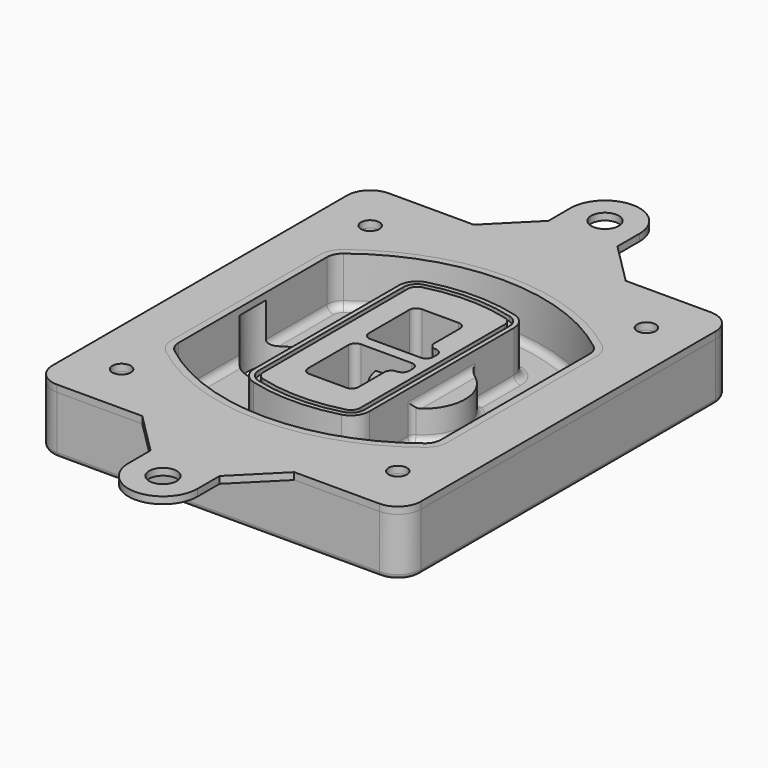
from build123d import *

# Parameters (mm, degrees)
F0_R      = 4
F1_DEPTH  = 25
F2_DEPTH  = 3
F3_DEPTH  = 18
F5_DEPTH  = 21
F6_DEPTH  = 2
F8_DEPTH  = 20
F9_DEPTH  = 16
F10_DEPTH = 25
F7_R      = 6
F7_R_2    = 4
F11_DEPTH = 6
F13_DEPTH = 9
F14_R     = 3
F15_R     = 2
F16_R     = 6
F16_R_2   = 4
F17_DEPTH = 3


# Not quite as in the source:
# - a feature names something its author has since deleted; it is built from what else it names


with BuildPart() as f1:
    # F0 (on Top) → F1 (new body)
    with BuildSketch(Plane.XY):
        with BuildLine():
            ThreePointArc((-80, -80), (-77.0710678119, -87.0710678119), (-70, -90))
            Line((-70, -90), (70, -90))
            ThreePointArc((70, -90), (77.0710678119, -87.0710678119), (80, -80))
            Line((80, -80), (80, 80))
            ThreePointArc((80, 80), (77.0710678119, 87.0710678119), (70, 90))
            Line((70, 90), (-70, 90))
            ThreePointArc((-70, 90), (-77.0710678119, 87.0710678119), (-80, 80))
            Line((-80, 80), (-80, -80))
        make_face()
        with Locations((-60, -67.5)):
            Circle(F0_R, mode=Mode.SUBTRACT)
        with Locations((60, -67.5)):
            Circle(F0_R, mode=Mode.SUBTRACT)
        with Locations((-60, 67.5)):
            Circle(F0_R, mode=Mode.SUBTRACT)
        with BuildLine():
            ThreePointArc((-64, 40.2934422872), (-62.5820384798, 46.4328484224), (-58.6153846154, 51.3286200352))
            ThreePointArc((-58.6153846154, 51.3286200352), (0, 71.5), (58.6153846154, 51.3286200352))
            ThreePointArc((58.6153846154, 51.3286200352), (62.5820384798, 46.4328484224), (64, 40.2934422872))
            Line((64, 40.2934422872), (64, -40.2934422872))
            ThreePointArc((64, -40.2934422872), (62.5820384798, -46.4328484224), (58.6153846154, -51.3286200352))
            ThreePointArc((58.6153846154, -51.3286200352), (0, -71.5), (-58.6153846154, -51.3286200352))
            ThreePointArc((-58.6153846154, -51.3286200352), (-62.5820384798, -46.4328484224), (-64, -40.2934422872))
            Line((-64, -40.2934422872), (-64, 40.2934422872))
        make_face(mode=Mode.SUBTRACT)
        with Locations((60, 67.5)):
            Circle(F0_R, mode=Mode.SUBTRACT)
        with BuildLine():
            ThreePointArc((58.6153846154, 51.3286200352), (0, 71.5), (-58.6153846154, 51.3286200352))
            ThreePointArc((-58.6153846154, 51.3286200352), (-62.5820384798, 46.4328484224), (-64, 40.2934422872))
            Line((-64, 40.2934422872), (-64, -40.2934422872))
            ThreePointArc((-64, -40.2934422872), (-62.5820384798, -46.4328484224), (-58.6153846154, -51.3286200352))
            ThreePointArc((-58.6153846154, -51.3286200352), (0, -71.5), (58.6153846154, -51.3286200352))
            ThreePointArc((58.6153846154, -51.3286200352), (62.5820384798, -46.4328484224), (64, -40.2934422872))
            Line((64, -40.2934422872), (64, 40.2934422872))
            ThreePointArc((64, 40.2934422872), (62.5820384798, 46.4328484224), (58.6153846154, 51.3286200352))
        make_face()
        with BuildLine():
            Line((-60, -40.2934422872), (-60, 40.2934422872))
            ThreePointArc((-60, 40.2934422872), (-58.9871703427, 44.6787323838), (-56.1538461538, 48.1757121072))
            ThreePointArc((-56.1538461538, 48.1757121072), (0, 67.5), (56.1538461538, 48.1757121072))
            ThreePointArc((56.1538461538, 48.1757121072), (58.9871703427, 44.6787323838), (60, 40.2934422872))
            Line((60, 40.2934422872), (60, -40.2934422872))
            ThreePointArc((60, -40.2934422872), (58.9871703427, -44.6787323838), (56.1538461538, -48.1757121072))
            ThreePointArc((56.1538461538, -48.1757121072), (0, -67.5), (-56.1538461538, -48.1757121072))
            ThreePointArc((-56.1538461538, -48.1757121072), (-58.9871703427, -44.6787323838), (-60, -40.2934422872))
        make_face(mode=Mode.SUBTRACT)
        with BuildLine():
            ThreePointArc((-56.1538461538, 48.1757121072), (-58.9871703427, 44.6787323838), (-60, 40.2934422872))
            Line((-60, 40.2934422872), (-60, -40.2934422872))
            ThreePointArc((-60, -40.2934422872), (-58.9871703427, -44.6787323838), (-56.1538461538, -48.1757121072))
            ThreePointArc((-56.1538461538, -48.1757121072), (0, -67.5), (56.1538461538, -48.1757121072))
            ThreePointArc((56.1538461538, -48.1757121072), (58.9871703427, -44.6787323838), (60, -40.2934422872))
            Line((60, -40.2934422872), (60, 40.2934422872))
            ThreePointArc((60, 40.2934422872), (58.9871703427, 44.6787323838), (56.1538461538, 48.1757121072))
            ThreePointArc((56.1538461538, 48.1757121072), (0, 67.5), (-56.1538461538, 48.1757121072))
        make_face()
        with BuildLine():
            ThreePointArc((54.3076923077, 45.8110311612), (56.2910192399, 43.3631453548), (57, 40.2934422872))
            Line((57, 40.2934422872), (57, -40.2934422872))
            ThreePointArc((57, -40.2934422872), (56.2910192399, -43.3631453548), (54.3076923077, -45.8110311612))
            ThreePointArc((54.3076923077, -45.8110311612), (0, -64.5), (-54.3076923077, -45.8110311612))
            ThreePointArc((-54.3076923077, -45.8110311612), (-56.2910192399, -43.3631453548), (-57, -40.2934422872))
            Line((-57, -40.2934422872), (-57, 40.2934422872))
            ThreePointArc((-57, 40.2934422872), (-56.2910192399, 43.3631453548), (-54.3076923077, 45.8110311612))
            ThreePointArc((-54.3076923077, 45.8110311612), (0, 64.5), (54.3076923077, 45.8110311612))
        make_face(mode=Mode.SUBTRACT)
        with BuildLine():
            Line((57, -40.2934422872), (57, 40.2934422872))
            ThreePointArc((57, 40.2934422872), (56.2910192399, 43.3631453548), (54.3076923077, 45.8110311612))
            ThreePointArc((54.3076923077, 45.8110311612), (0, 64.5), (-54.3076923077, 45.8110311612))
            ThreePointArc((-54.3076923077, 45.8110311612), (-56.2910192399, 43.3631453548), (-57, 40.2934422872))
            Line((-57, 40.2934422872), (-57, -40.2934422872))
            ThreePointArc((-57, -40.2934422872), (-56.2910192399, -43.3631453548), (-54.3076923077, -45.8110311612))
            ThreePointArc((-54.3076923077, -45.8110311612), (0, -64.5), (54.3076923077, -45.8110311612))
            ThreePointArc((54.3076923077, -45.8110311612), (56.2910192399, -43.3631453548), (57, -40.2934422872))
        make_face()
    extrude(amount=-F1_DEPTH)

    # F0 (on Top) → F2 (join)
    with BuildSketch(Plane.XY):
        with BuildLine():
            ThreePointArc((-56.1538461538, 48.1757121072), (-58.9871703427, 44.6787323838), (-60, 40.2934422872))
            Line((-60, 40.2934422872), (-60, -40.2934422872))
            ThreePointArc((-60, -40.2934422872), (-58.9871703427, -44.6787323838), (-56.1538461538, -48.1757121072))
            ThreePointArc((-56.1538461538, -48.1757121072), (0, -67.5), (56.1538461538, -48.1757121072))
            ThreePointArc((56.1538461538, -48.1757121072), (58.9871703427, -44.6787323838), (60, -40.2934422872))
            Line((60, -40.2934422872), (60, 40.2934422872))
            ThreePointArc((60, 40.2934422872), (58.9871703427, 44.6787323838), (56.1538461538, 48.1757121072))
            ThreePointArc((56.1538461538, 48.1757121072), (0, 67.5), (-56.1538461538, 48.1757121072))
        make_face()
        with BuildLine():
            ThreePointArc((54.3076923077, 45.8110311612), (56.2910192399, 43.3631453548), (57, 40.2934422872))
            Line((57, 40.2934422872), (57, -40.2934422872))
            ThreePointArc((57, -40.2934422872), (56.2910192399, -43.3631453548), (54.3076923077, -45.8110311612))
            ThreePointArc((54.3076923077, -45.8110311612), (0, -64.5), (-54.3076923077, -45.8110311612))
            ThreePointArc((-54.3076923077, -45.8110311612), (-56.2910192399, -43.3631453548), (-57, -40.2934422872))
            Line((-57, -40.2934422872), (-57, 40.2934422872))
            ThreePointArc((-57, 40.2934422872), (-56.2910192399, 43.3631453548), (-54.3076923077, 45.8110311612))
            ThreePointArc((-54.3076923077, 45.8110311612), (0, 64.5), (54.3076923077, 45.8110311612))
        make_face(mode=Mode.SUBTRACT)
    extrude(amount=F2_DEPTH)

    # F0 (on Top) → F3 (cut)
    with BuildSketch(Plane.XY):
        with BuildLine():
            Line((57, -40.2934422872), (57, 40.2934422872))
            ThreePointArc((57, 40.2934422872), (56.2910192399, 43.3631453548), (54.3076923077, 45.8110311612))
            ThreePointArc((54.3076923077, 45.8110311612), (0, 64.5), (-54.3076923077, 45.8110311612))
            ThreePointArc((-54.3076923077, 45.8110311612), (-56.2910192399, 43.3631453548), (-57, 40.2934422872))
            Line((-57, 40.2934422872), (-57, -40.2934422872))
            ThreePointArc((-57, -40.2934422872), (-56.2910192399, -43.3631453548), (-54.3076923077, -45.8110311612))
            ThreePointArc((-54.3076923077, -45.8110311612), (0, -64.5), (54.3076923077, -45.8110311612))
            ThreePointArc((54.3076923077, -45.8110311612), (56.2910192399, -43.3631453548), (57, -40.2934422872))
        make_face()
    extrude(amount=-F3_DEPTH, mode=Mode.SUBTRACT)

    # F4 (on face) → F5 (join, through all)
    with BuildSketch(Plane.XY.offset(3)):
        with BuildLine():
            ThreePointArc((-25, -39.2465276821), (-23.3511545998, -44.1109737193), (-19.0842911877, -46.9702398883))
            ThreePointArc((-19.0842911877, -46.9702398883), (0, -49.5), (19.0842911877, -46.9702398883))
            ThreePointArc((19.0842911877, -46.9702398883), (23.3511545998, -44.1109737193), (25, -39.2465276821))
            Line((25, -39.2465276821), (25, 39.2465276821))
            ThreePointArc((25, 39.2465276821), (23.3511545998, 44.1109737193), (19.0842911877, 46.9702398883))
            ThreePointArc((19.0842911877, 46.9702398883), (0, 49.5), (-19.0842911877, 46.9702398883))
            ThreePointArc((-19.0842911877, 46.9702398883), (-23.3511545998, 44.1109737193), (-25, 39.2465276821))
            Line((-25, 39.2465276821), (-25, -39.2465276821))
        make_face()
        with BuildLine():
            ThreePointArc((18.5632183908, 45.0393118368), (21.7633659499, 42.89486221), (23, 39.2465276821))
            Line((23, 39.2465276821), (23, -39.2465276821))
            ThreePointArc((23, -39.2465276821), (21.7633659499, -42.89486221), (18.5632183908, -45.0393118368))
            ThreePointArc((18.5632183908, -45.0393118368), (0, -47.5), (-18.5632183908, -45.0393118368))
            ThreePointArc((-18.5632183908, -45.0393118368), (-21.7633659499, -42.89486221), (-23, -39.2465276821))
            Line((-23, -39.2465276821), (-23, 39.2465276821))
            ThreePointArc((-23, 39.2465276821), (-21.7633659499, 42.89486221), (-18.5632183908, 45.0393118368))
            ThreePointArc((-18.5632183908, 45.0393118368), (0, 47.5), (18.5632183908, 45.0393118368))
        make_face(mode=Mode.SUBTRACT)
        with BuildLine():
            Line((23, -39.2465276821), (23, 39.2465276821))
            ThreePointArc((23, 39.2465276821), (21.7633659499, 42.89486221), (18.5632183908, 45.0393118368))
            ThreePointArc((18.5632183908, 45.0393118368), (0, 47.5), (-18.5632183908, 45.0393118368))
            ThreePointArc((-18.5632183908, 45.0393118368), (-21.7633659499, 42.89486221), (-23, 39.2465276821))
            Line((-23, 39.2465276821), (-23, -39.2465276821))
            ThreePointArc((-23, -39.2465276821), (-21.7633659499, -42.89486221), (-18.5632183908, -45.0393118368))
            ThreePointArc((-18.5632183908, -45.0393118368), (0, -47.5), (18.5632183908, -45.0393118368))
            ThreePointArc((18.5632183908, -45.0393118368), (21.7633659499, -42.89486221), (23, -39.2465276821))
        make_face()
        with BuildLine():
            ThreePointArc((18.0421455939, 43.1083837852), (20.1755772999, 41.6787507007), (21, 39.2465276821))
            Line((21, 39.2465276821), (21, -39.2465276821))
            ThreePointArc((21, -39.2465276821), (20.1755772999, -41.6787507007), (18.0421455939, -43.1083837852))
            ThreePointArc((18.0421455939, -43.1083837852), (0, -45.5), (-18.0421455939, -43.1083837852))
            ThreePointArc((-18.0421455939, -43.1083837852), (-20.1755772999, -41.6787507007), (-21, -39.2465276821))
            Line((-21, -39.2465276821), (-21, 39.2465276821))
            ThreePointArc((-21, 39.2465276821), (-20.1755772999, 41.6787507007), (-18.0421455939, 43.1083837852))
            ThreePointArc((-18.0421455939, 43.1083837852), (0, 45.5), (18.0421455939, 43.1083837852))
        make_face(mode=Mode.SUBTRACT)
        with BuildLine():
            Line((21, -39.2465276821), (21, 39.2465276821))
            ThreePointArc((21, 39.2465276821), (20.1755772999, 41.6787507007), (18.0421455939, 43.1083837852))
            ThreePointArc((18.0421455939, 43.1083837852), (0, 45.5), (-18.0421455939, 43.1083837852))
            ThreePointArc((-18.0421455939, 43.1083837852), (-20.1755772999, 41.6787507007), (-21, 39.2465276821))
            Line((-21, 39.2465276821), (-21, -39.2465276821))
            ThreePointArc((-21, -39.2465276821), (-20.1755772999, -41.6787507007), (-18.0421455939, -43.1083837852))
            ThreePointArc((-18.0421455939, -43.1083837852), (0, -45.5), (18.0421455939, -43.1083837852))
            ThreePointArc((18.0421455939, -43.1083837852), (20.1755772999, -41.6787507007), (21, -39.2465276821))
        make_face()
        with BuildLine():
            Line((-8, -2.5), (14, -2.5))
            ThreePointArc((14, -2.5), (16.1213203436, -3.3786796564), (17, -5.5))
            Line((17, -5.5), (17, -7.5))
            ThreePointArc((17, -7.5), (16.1213203436, -9.6213203436), (14, -10.5))
            ThreePointArc((14, -10.5), (11.8786796564, -11.3786796564), (11, -13.5))
            Line((11, -13.5), (11, -27.5))
            ThreePointArc((11, -27.5), (10.1213203436, -29.6213203436), (8, -30.5))
            Line((8, -30.5), (-8, -30.5))
            ThreePointArc((-8, -30.5), (-10.1213203436, -29.6213203436), (-11, -27.5))
            Line((-11, -27.5), (-11, -5.5))
            ThreePointArc((-11, -5.5), (-10.1213203436, -3.3786796564), (-8, -2.5))
        make_face(mode=Mode.SUBTRACT)
        with BuildLine():
            ThreePointArc((-8, 2.5), (-10.1213203436, 3.3786796564), (-11, 5.5))
            Line((-11, 5.5), (-11, 27.5))
            ThreePointArc((-11, 27.5), (-10.1213203436, 29.6213203436), (-8, 30.5))
            Line((-8, 30.5), (8, 30.5))
            ThreePointArc((8, 30.5), (10.1213203436, 29.6213203436), (11, 27.5))
            Line((11, 27.5), (11, 13.5))
            ThreePointArc((11, 13.5), (11.8786796564, 11.3786796564), (14, 10.5))
            ThreePointArc((14, 10.5), (16.1213203436, 9.6213203436), (17, 7.5))
            Line((17, 7.5), (17, 5.5))
            ThreePointArc((17, 5.5), (16.1213203436, 3.3786796564), (14, 2.5))
            Line((14, 2.5), (-8, 2.5))
        make_face(mode=Mode.SUBTRACT)
    extrude(amount=-F5_DEPTH)

    # F4 (on face) → F6 (cut)
    with BuildSketch(Plane.XY.offset(3)):
        with BuildLine():
            Line((23, -39.2465276821), (23, 39.2465276821))
            ThreePointArc((23, 39.2465276821), (21.7633659499, 42.89486221), (18.5632183908, 45.0393118368))
            ThreePointArc((18.5632183908, 45.0393118368), (0, 47.5), (-18.5632183908, 45.0393118368))
            ThreePointArc((-18.5632183908, 45.0393118368), (-21.7633659499, 42.89486221), (-23, 39.2465276821))
            Line((-23, 39.2465276821), (-23, -39.2465276821))
            ThreePointArc((-23, -39.2465276821), (-21.7633659499, -42.89486221), (-18.5632183908, -45.0393118368))
            ThreePointArc((-18.5632183908, -45.0393118368), (0, -47.5), (18.5632183908, -45.0393118368))
            ThreePointArc((18.5632183908, -45.0393118368), (21.7633659499, -42.89486221), (23, -39.2465276821))
        make_face()
        with BuildLine():
            ThreePointArc((18.0421455939, 43.1083837852), (20.1755772999, 41.6787507007), (21, 39.2465276821))
            Line((21, 39.2465276821), (21, -39.2465276821))
            ThreePointArc((21, -39.2465276821), (20.1755772999, -41.6787507007), (18.0421455939, -43.1083837852))
            ThreePointArc((18.0421455939, -43.1083837852), (0, -45.5), (-18.0421455939, -43.1083837852))
            ThreePointArc((-18.0421455939, -43.1083837852), (-20.1755772999, -41.6787507007), (-21, -39.2465276821))
            Line((-21, -39.2465276821), (-21, 39.2465276821))
            ThreePointArc((-21, 39.2465276821), (-20.1755772999, 41.6787507007), (-18.0421455939, 43.1083837852))
            ThreePointArc((-18.0421455939, 43.1083837852), (0, 45.5), (18.0421455939, 43.1083837852))
        make_face(mode=Mode.SUBTRACT)
    extrude(amount=-F6_DEPTH, mode=Mode.SUBTRACT)

    # F7 (on face) → F8 (join)
    with BuildSketch(Plane(origin=(0, 0, -25), x_dir=(1, 0, 0), z_dir=(0, 0, -1))):
        with BuildLine():
            ThreePointArc((3.28842436, 0), (16.7567035675, 13.4682792075), (30.224982775, 0))
            Line((30.224982775, 0), (35.224982775, 0))
            ThreePointArc((35.224982775, 0), (16.7567035675, 18.4682792075), (-1.71157564, 0))
            Line((-1.71157564, 0), (3.28842436, 0))
        make_face()
        with BuildLine():
            Line((3.28842436, 0), (30.224982775, 0))
            ThreePointArc((30.224982775, 0), (16.7567035675, 13.4682792075), (3.28842436, 0))
        make_face()
        with BuildLine():
            ThreePointArc((3.28842436, 0), (16.7567035675, -13.4682792075), (30.224982775, 0))
            Line((30.224982775, 0), (3.28842436, 0))
        make_face()
        with BuildLine():
            Line((35.224982775, 0), (30.224982775, 0))
            ThreePointArc((30.224982775, 0), (16.7567035675, -13.4682792075), (3.28842436, 0))
            Line((3.28842436, 0), (-1.71157564, 0))
            ThreePointArc((-1.71157564, 0), (16.7567035675, -18.4682792075), (35.224982775, 0))
        make_face()
    extrude(amount=-F8_DEPTH)

    # F7 (on face) → F9 (cut)
    with BuildSketch(Plane(origin=(0, 0, -25), x_dir=(1, 0, 0), z_dir=(0, 0, -1))):
        with BuildLine():
            Line((3.28842436, 0), (30.224982775, 0))
            ThreePointArc((30.224982775, 0), (16.7567035675, 13.4682792075), (3.28842436, 0))
        make_face()
        with BuildLine():
            ThreePointArc((3.28842436, 0), (16.7567035675, -13.4682792075), (30.224982775, 0))
            Line((30.224982775, 0), (3.28842436, 0))
        make_face()
    extrude(amount=-F9_DEPTH, mode=Mode.SUBTRACT)

    # F7 (on face) → F10 (cut)
    with BuildSketch(Plane(origin=(0, 0, -25), x_dir=(1, 0, 0), z_dir=(0, 0, -1))):
        with BuildLine():
            Line((-59.0318229325, 0), (-32.0952645175, 0))
            ThreePointArc((-32.0952645175, 0), (-45.563543725, 13.4682792075), (-59.0318229325, 0))
        make_face()
        with BuildLine():
            ThreePointArc((-59.0318229325, 0), (-45.563543725, -13.4682792075), (-32.0952645175, 0))
            Line((-32.0952645175, 0), (-59.0318229325, 0))
        make_face()
    extrude(amount=-F10_DEPTH, mode=Mode.SUBTRACT)

    # F7 (on face) → F11 (cut)
    with BuildSketch(Plane(origin=(0, 0, -25), x_dir=(1, 0, 0), z_dir=(0, 0, -1))):
        with Locations((60, -67.5)):
            Circle(F7_R)
        with Locations((60, -67.5)):
            Circle(F7_R_2, mode=Mode.SUBTRACT)
        with Locations((-60, -67.5)):
            Circle(F7_R)
        with Locations((-60, -67.5)):
            Circle(F7_R_2, mode=Mode.SUBTRACT)
        with Locations((-60, 67.5)):
            Circle(F7_R)
        with Locations((-60, 67.5)):
            Circle(F7_R_2, mode=Mode.SUBTRACT)
        with Locations((60, 67.5)):
            Circle(F7_R)
        with Locations((60, 67.5)):
            Circle(F7_R_2, mode=Mode.SUBTRACT)
    extrude(amount=-F11_DEPTH, mode=Mode.SUBTRACT)

    # F12 (on face) → F13 (cut, through all)
    with BuildSketch(Plane(origin=(0, 0, -9), x_dir=(1, 0, 0), z_dir=(0, 0, -1))):
        with BuildLine():
            Line((11, 13.5), (11, 17.5481537753))
            ThreePointArc((11, 17.5481537753), (2.5696536419, 11.8239143813), (-1.5415842455, 2.5))
            Line((-1.5415842455, 2.5), (3.5224848595, 2.5))
            ThreePointArc((3.5224848595, 2.5), (6.1857188154, 8.3455872281), (11.2536447004, 12.2927168648))
            ThreePointArc((11.2536447004, 12.2927168648), (11.0640958889, 12.8831798879), (11, 13.5))
        make_face()
        with BuildLine():
            ThreePointArc((11.2536447004, -12.2927168648), (6.1857188154, -8.3455872281), (3.5224848595, -2.5))
            Line((3.5224848595, -2.5), (-1.5415842455, -2.5))
            ThreePointArc((-1.5415842455, -2.5), (2.5696536419, -11.8239143813), (11, -17.5481537753))
            Line((11, -17.5481537753), (11, -13.5))
            ThreePointArc((11, -13.5), (11.0640958889, -12.8831798879), (11.2536447004, -12.2927168648))
        make_face()
        with BuildLine():
            ThreePointArc((11.2536447004, 12.2927168648), (6.1857188154, 8.3455872281), (3.5224848595, 2.5))
            Line((3.5224848595, 2.5), (14, 2.5))
            ThreePointArc((14, 2.5), (16.1213203436, 3.3786796564), (17, 5.5))
            Line((17, 5.5), (17, 7.5))
            ThreePointArc((17, 7.5), (16.1213203436, 9.6213203436), (14, 10.5))
            ThreePointArc((14, 10.5), (12.3601599782, 10.9878446101), (11.2536447004, 12.2927168648))
        make_face()
        with BuildLine():
            Line((14, -2.5), (3.5224848595, -2.5))
            ThreePointArc((3.5224848595, -2.5), (6.1857188154, -8.3455872281), (11.2536447004, -12.2927168648))
            ThreePointArc((11.2536447004, -12.2927168648), (12.3601599782, -10.9878446101), (14, -10.5))
            ThreePointArc((14, -10.5), (16.1213203436, -9.6213203436), (17, -7.5))
            Line((17, -7.5), (17, -5.5))
            ThreePointArc((17, -5.5), (16.1213203436, -3.3786796564), (14, -2.5))
        make_face()
    extrude(amount=F13_DEPTH, mode=Mode.SUBTRACT)

    # F14
    f14_edges = [f1.edges().sort_by_distance(p)[0] for p in [
        (-57, -23.703476, -18),
        (-57, 23.703476, -18),
        (25, 0, -5),
        (25, 16.526506, -11.5),
        (25, -16.526506, -11.5),
        (25, -27.886517, -18),
        (35.224983, 0, -18),
    ]]
    fillet(f14_edges, radius=F14_R)

    # F15
    f15_edges = [f1.edges().sort_by_distance(p)[0] for p in [
        (0, -90, -25),
    ]]
    fillet(f15_edges, radius=F15_R)


with BuildPart() as f17:
    # F16 (on face) → F17 (new body, through all)
    with BuildSketch(Plane.XY):
        with BuildLine():
            Line((-15, 120), (-15, 108))
            Line((-15, 108), (-33, 90))
            Line((-33, 90), (33, 90))
            Line((33, 90), (15, 108))
            Line((15, 108), (15, 120))
            ThreePointArc((15, 120), (0, 135), (-15, 120))
        make_face()
        with Locations((0, 120)):
            Circle(F16_R, mode=Mode.SUBTRACT)
        with BuildLine():
            Line((33, 90), (-33, 90))
            Line((-33, 90), (-70, 90))
            ThreePointArc((-70, 90), (-77.0710678119, 87.0710678119), (-80, 80))
            Line((-80, 80), (-80, 0))
            Line((-80, 0), (-60, 0))
            Line((-60, 0), (-60, 40.2934422872))
            ThreePointArc((-60, 40.2934422872), (-58.9871703427, 44.6787323838), (-56.1538461538, 48.1757121072))
            ThreePointArc((-56.1538461538, 48.1757121072), (0, 67.5), (56.1538461538, 48.1757121072))
            ThreePointArc((56.1538461538, 48.1757121072), (58.9871703427, 44.6787323838), (60, 40.2934422872))
            Line((60, 40.2934422872), (60, 0))
            Line((60, 0), (80, 0))
            Line((80, 0), (80, 80))
            ThreePointArc((80, 80), (77.0710678119, 87.0710678119), (70, 90))
            Line((70, 90), (33, 90))
        make_face()
        with Locations((-60, 67.5)):
            Circle(F16_R_2, mode=Mode.SUBTRACT)
        with Locations((60, 67.5)):
            Circle(F16_R_2, mode=Mode.SUBTRACT)
        with BuildLine():
            Line((-60, 0), (-80, 0))
            Line((-80, 0), (-80, -80))
            ThreePointArc((-80, -80), (-77.0710678119, -87.0710678119), (-70, -90))
            Line((-70, -90), (-33, -90))
            Line((-33, -90), (33, -90))
            Line((33, -90), (70, -90))
            ThreePointArc((70, -90), (77.0710678119, -87.0710678119), (80, -80))
            Line((80, -80), (80, 0))
            Line((80, 0), (60, 0))
            Line((60, 0), (60, -40.2934422872))
            ThreePointArc((60, -40.2934422872), (58.9871703427, -44.6787323838), (56.1538461538, -48.1757121072))
            ThreePointArc((56.1538461538, -48.1757121072), (0, -67.5), (-56.1538461538, -48.1757121072))
            ThreePointArc((-56.1538461538, -48.1757121072), (-58.9871703427, -44.6787323838), (-60, -40.2934422872))
            Line((-60, -40.2934422872), (-60, 0))
        make_face()
        with Locations((-60, -67.5)):
            Circle(F16_R_2, mode=Mode.SUBTRACT)
        with Locations((60, -67.5)):
            Circle(F16_R_2, mode=Mode.SUBTRACT)
        with BuildLine():
            Line((33, -90), (-33, -90))
            Line((-33, -90), (-15, -108))
            Line((-15, -108), (-15, -120))
            ThreePointArc((-15, -120), (0, -135), (15, -120))
            Line((15, -120), (15, -108))
            Line((15, -108), (33, -90))
        make_face()
        with Locations((0, -120)):
            Circle(F16_R, mode=Mode.SUBTRACT)
    extrude(amount=F17_DEPTH)


solid = Compound([f1.part, f17.part])
